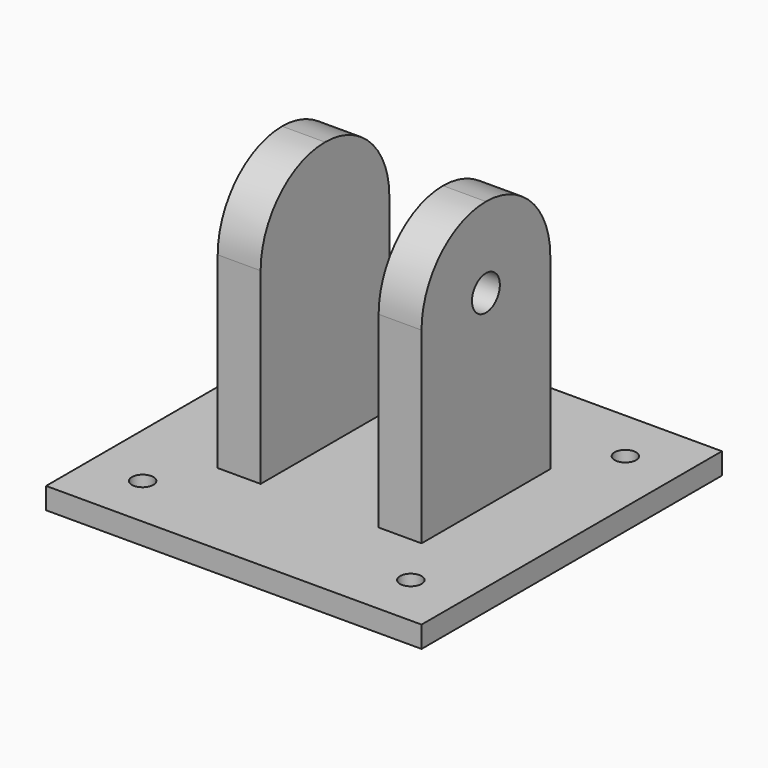
from build123d import *

# Parameters (mm, degrees)
F0_W     = 70
F0_H     = 70
F1_DEPTH = 4
F2_W     = 8
F2_H     = 30
F3_DEPTH = 50
F4_R     = 14.99999
F7_D     = 6.5
F7_DEPTH = 15
F7_TIP   = 1.9527970118
F8_D     = 4
F8_DEPTH = 15
F8_TIP   = 1.2017212381


# Not quite as in the source:
# - a fillet or chamfer is up to 0.001 mm smaller than in the source, because OpenCascade refuses the exact size


with BuildPart() as f1:
    # F0 (on Top) → F1 (new body)
    with BuildSketch(Plane.XY):
        with Locations((1.0378739359, 35)):
            Rectangle(F0_W, F0_H)
    extrude(amount=F1_DEPTH)

    # F2 (on face) → F3 (join)
    with BuildSketch(Plane.XY.offset(4)):
        with Locations((-13.9621260641, 35)):
            Rectangle(F2_W, F2_H)
        with Locations((16.0378739359, 35)):
            Rectangle(F2_W, F2_H)
    extrude(amount=F3_DEPTH)

    # F4 (radius 15 in the source; OpenCascade refuses exactly that, so slightly less here)
    f4_edges = [f1.edges().sort_by_distance(p)[0] for p in [
        (-13.962126, 20, 54),
        (-13.962126, 50, 54),
        (16.037874, 20, 54),
        (16.037874, 50, 54),
    ]]
    fillet(f4_edges, radius=F4_R)

    # F7
    with Locations(Plane.YZ.offset(20.0378739359)):
        with Locations((35, 39)):
            Hole(F7_D / 2, depth=F7_DEPTH)
            with Locations((0, 0, -(F7_DEPTH + F7_TIP / 2))):  # 118° drill point
                Cone(0, F7_D / 2, F7_TIP, mode=Mode.SUBTRACT)

    # F8
    with Locations(Plane.XY.offset(4)):
        with Locations((-23.9621260641, 10), (26.0378739359, 10), (26.0378739359, 60), (-23.9621260641, 60)):
            Hole(F8_D / 2, depth=F8_DEPTH)
            with Locations((0, 0, -(F8_DEPTH + F8_TIP / 2))):  # 118° drill point
                Cone(0, F8_D / 2, F8_TIP, mode=Mode.SUBTRACT)


solid = f1.part
